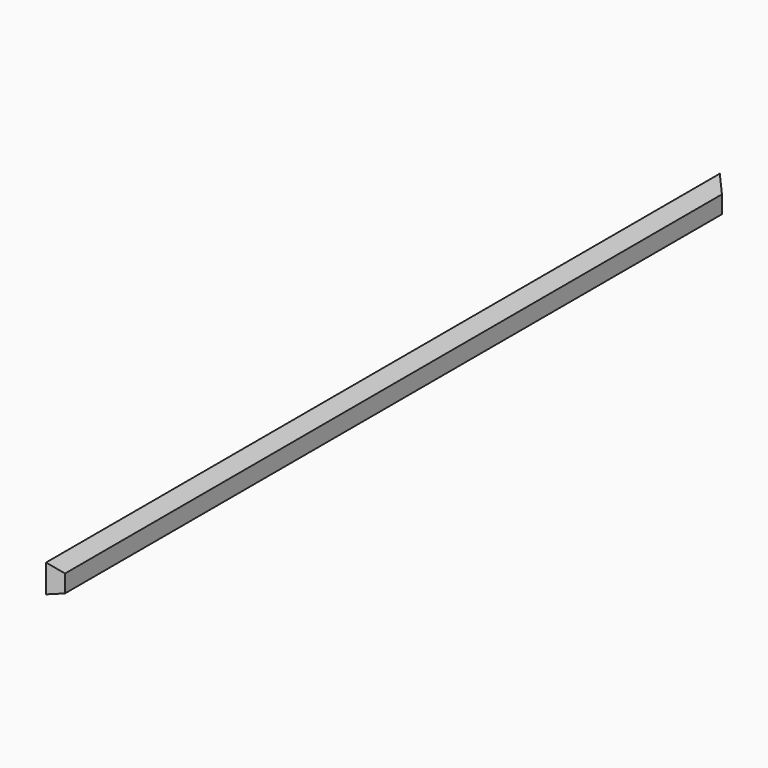
from build123d import *

# Parameters (mm, degrees)
F0_W     = 1524
F0_H     = 50.8
F1_DEPTH = 19.05
F3_DEPTH = 50.801
F5_DEPTH = 1524.001


# Not quite as in the source:
# - a pattern or mirror of a feature is missing from the dataset's text; its kind, count and spacing are read off the source's solid


with BuildPart() as f1:
    # F0 (on Right) → F1 (new body)
    with BuildSketch(Plane.YZ):
        Rectangle(F0_W, F0_H)
    extrude(amount=F1_DEPTH)

    # F2 (on face) → F3 (cut, through all)
    with BuildSketch(Plane.XY.offset(25.4)):
        Polygon((19.05, 762), (0, 762), (19.05, 742.95), align=None)
    f3 = extrude(amount=-F3_DEPTH, mode=Mode.SUBTRACT)

    # F3_copies: F3 across plane
    add(f3.mirror(Plane(origin=(0, 0, 0), x_dir=(0, 0, -1), z_dir=(0, -1, 0))), mode=Mode.SUBTRACT)

    # F4 (on face) → F5 (cut, through all)
    with BuildSketch(Plane.XZ.offset(762)):
        Polygon((19.05, 25.4), (0, 25.4), (19.05, 6.35), align=None)
    extrude(amount=-F5_DEPTH, mode=Mode.SUBTRACT)


solid = f1.part
